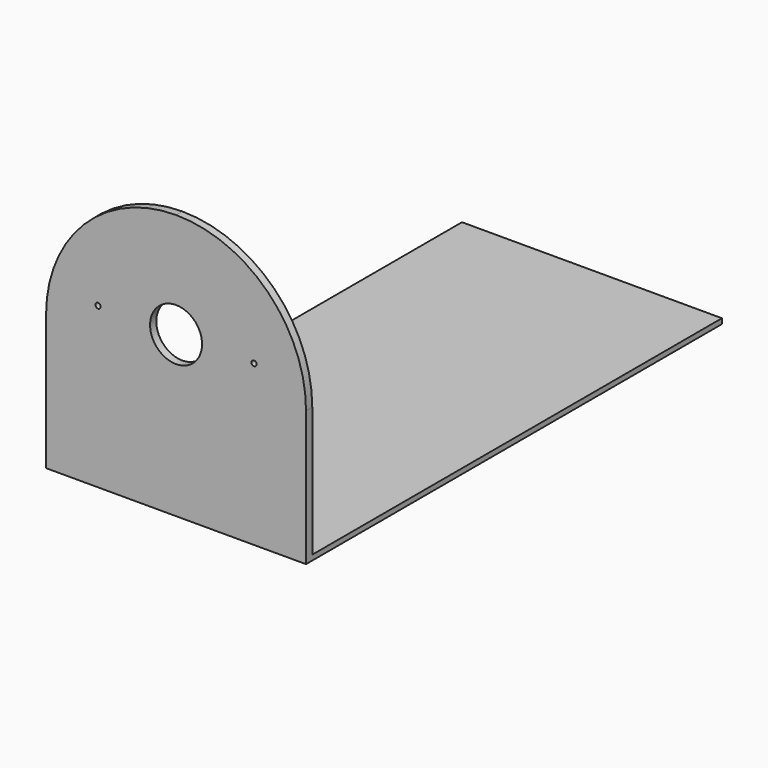
from build123d import *

# Parameters (mm, degrees)
F0_W     = 100
F0_H     = 200
F1_DEPTH = 2
F2_W     = 100
F2_H     = 3
F3_DEPTH = 100
F4_R     = 49.99999
F5_R     = 10
F6_DEPTH = 25
F5_R_2   = 1
F7_DEPTH = 25


# Not quite as in the source:
# - a fillet or chamfer is up to 0.001 mm smaller than in the source, because OpenCascade refuses the exact size


with BuildPart() as f1:
    # F0 (on Top) → F1 (new body)
    with BuildSketch(Plane.XY):
        Rectangle(F0_W, F0_H)
    extrude(amount=F1_DEPTH)

    # F2 (on face) → F3 (join)
    with BuildSketch(Plane.XY.offset(2)):
        with Locations((0, -98.5)):
            Rectangle(F2_W, F2_H)
    extrude(amount=F3_DEPTH)

    # F4 (radius 50 in the source; OpenCascade refuses exactly that, so slightly less here)
    f4_edges = [f1.edges().sort_by_distance(p)[0] for p in [
        (-50, -98.5, 102),
        (50, -98.5, 102),
    ]]
    fillet(f4_edges, radius=F4_R)

    # F5 (on face) → F6 (cut)
    with BuildSketch(Plane.XZ.offset(100)):
        with Locations((0, 61.5095198154)):
            Circle(F5_R)
    extrude(amount=-F6_DEPTH, mode=Mode.SUBTRACT)

    # F5 (on face) → F7 (cut)
    with BuildSketch(Plane.XZ.offset(100)):
        with Locations((0, 61.5095198154)):
            Circle(F5_R)
        with Locations((30, 61.5095198154)):
            Circle(F5_R_2)
        with Locations((-30, 61.5095198154)):
            Circle(F5_R_2)
    extrude(amount=-F7_DEPTH, mode=Mode.SUBTRACT)


solid = f1.part
